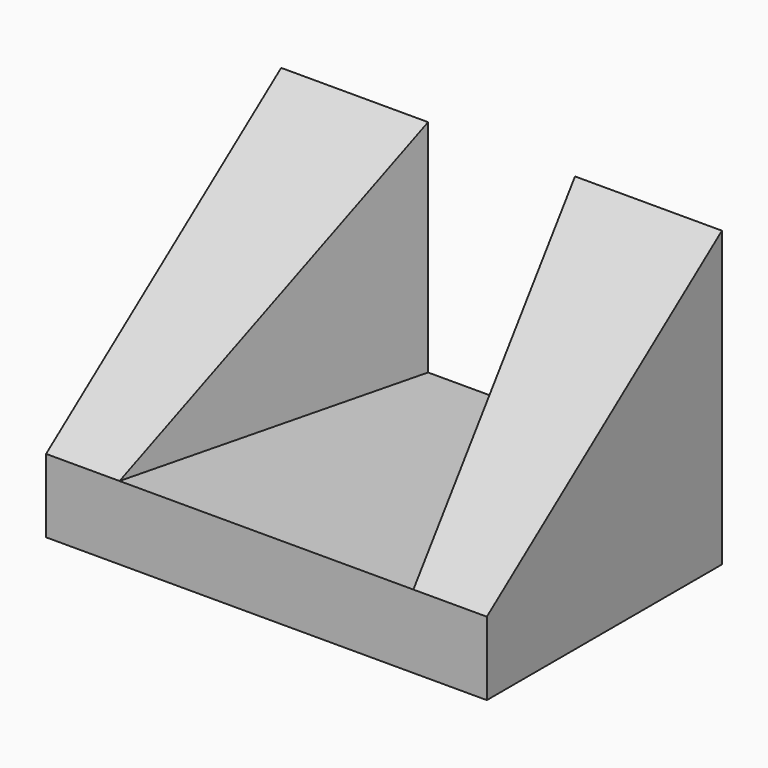
from build123d import *

# Parameters (mm, degrees)
F0_W     = 60
F0_H     = 40
F1_DEPTH = 40
F3_DEPTH = 30
F4_SIZE2 = 39.99999
F4_SIZE  = 29.99999


# Not quite as in the source:
# - a fillet or chamfer is up to 0.001 mm smaller than in the source, because OpenCascade refuses the exact size


with BuildPart() as f1:
    # F0 (on Top) → F1 (new body)
    with BuildSketch(Plane.XY):
        with Locations((0, 20)):
            Rectangle(F0_W, F0_H)
    extrude(amount=F1_DEPTH)

    # F2 (on face) → F3 (cut)
    with BuildSketch(Plane.XY.offset(40)):
        Polygon((-10, 40), (-20, 0), (20, 0), (10, 40), align=None)
    extrude(amount=-F3_DEPTH, mode=Mode.SUBTRACT)

    # F4 (size 30 and 40 in the source; OpenCascade refuses exactly that, so slightly less here)
    f4_edges = [f1.edges().sort_by_distance(p)[0] for p in [
        (-25, 0, 40),
        (25, 0, 40),
    ]]
    f4_side = f1.faces().sort_by_distance((0, 0, 0.72111))[0]
    chamfer(f4_edges, length=F4_SIZE, length2=F4_SIZE2, reference=f4_side)


solid = f1.part
